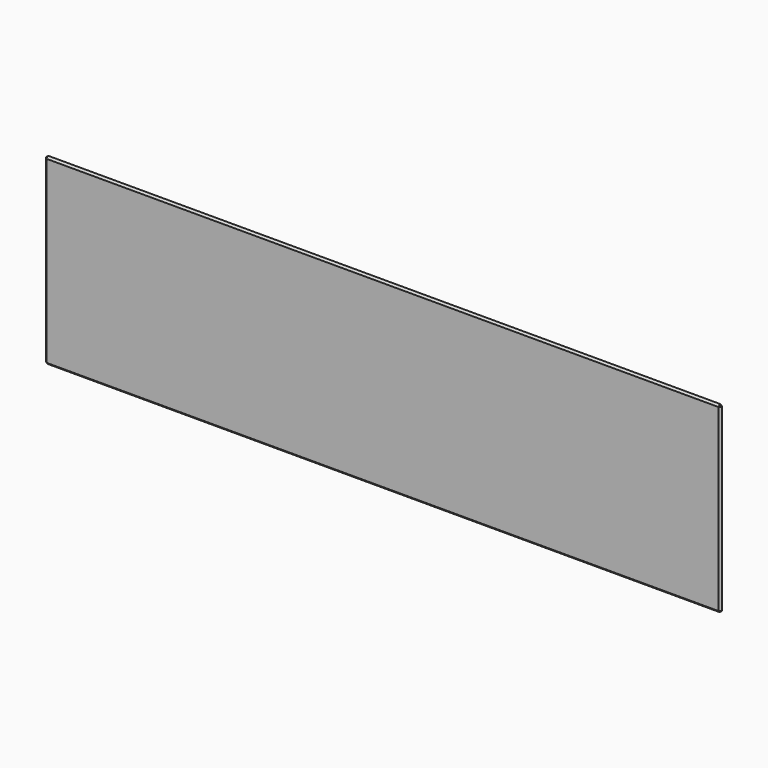
from build123d import *

# Parameters (mm, degrees)
F0_W     = 350
F0_H     = 95
F1_DEPTH = 2
F2_SIZE  = 0.99999


# Not quite as in the source:
# - a fillet or chamfer is up to 0.001 mm smaller than in the source, because OpenCascade refuses the exact size


with BuildPart() as f1:
    # F0 (on Front) → F1 (new body)
    with BuildSketch(Plane.XZ):
        Rectangle(F0_W, F0_H)
    extrude(amount=F1_DEPTH)

    # F2 (size 1 in the source; OpenCascade refuses exactly that, so slightly less here)
    f2_edges = [f1.edges().sort_by_distance(p)[0] for p in [
        (-175, 0, 0),
        (0, 0, 47.5),
        (0, -2, 47.5),
        (-175, -2, 0),
        (175, 0, 0),
        (0, 0, -47.5),
        (0, -2, -47.5),
        (175, -2, 0),
        (175, -1, -47.5),
        (175, -1, 47.5),
        (-175, -1, 47.5),
        (-175, -1, -47.5),
    ]]
    chamfer(f2_edges, length=F2_SIZE)


solid = f1.part
